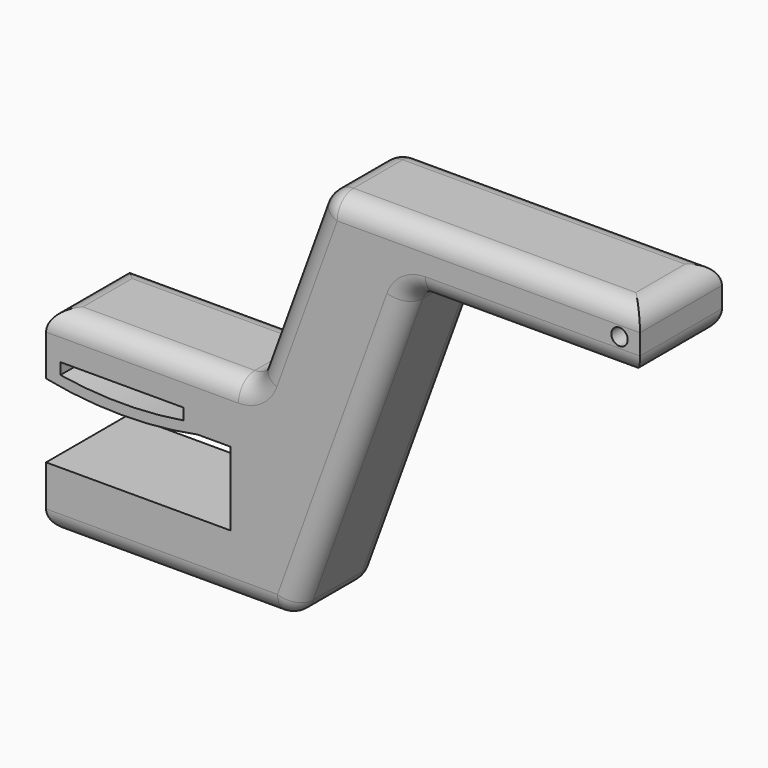
from build123d import *

# Parameters (mm, degrees)
F1_DEPTH = 25
F2_F1_R  = 5
F2_F2_R  = 5
F3_R     = 2
F4_DEPTH = 25


with BuildPart() as f1:
    # F0 (on Front) → F1 (new body)
    with BuildSketch(Plane.XZ):
        with BuildLine():
            Line((45, 15), (0, 15))
            Line((0, 15), (0, 0))
            Line((0, 0), (60, 0))
            Line((60, 0), (89.1176187413, 80))
            Line((89.1176187413, 80), (145, 80))
            Line((145, 80), (145, 95))
            Line((145, 95), (67.5712870168, 95))
            Line((67.5712870168, 95), (50.4646860063, 48))
            Line((50.4646860063, 48), (0, 48))
            Line((0, 48), (0, 33))
            ThreePointArc((0, 33), (18.5, 31.181274943), (37, 33))
            Line((37, 33), (45, 33))
            Line((45, 33), (45, 15))
        make_face()
        with BuildLine():
            ThreePointArc((33.5, 34.9055936253), (18.5, 33.681274943), (3.5, 34.9055936253))
            Line((3.5, 34.9055936253), (3.5, 37.681274943))
            Line((3.5, 37.681274943), (33.5, 37.681274943))
            Line((33.5, 37.681274943), (33.5, 34.9055936253))
        make_face(mode=Mode.SUBTRACT)
    extrude(amount=F1_DEPTH)

    # F2: fillet of radius 5 on 16 edges, made by hand

    # F2_f1
    f2_f1_edges = [f1.edges().sort_by_distance(p)[0] for p in [
        (89.1176187413, -12.5, 80),
        (50.4646860063, -12.5, 48),
    ]]
    fillet(f2_f1_edges, radius=F2_F1_R)

    # F2_f2
    f2_f2_edges = [f1.edges().sort_by_distance(p)[0] for p in [
        (60, -12.5, 0),
        (67.5712870168, -12.5, 95),
        (145, -12.5, 95),
        (145, -12.5, 80),
        (0, -12.5, 48),
        (0, -12.5, 0),
        (118.8093282162, -25, 80),
        (73.9600966642, 0, 38.3550503583),
        (106.2856435084, -25, 95),
        (59.616699218, -25, 73.1449496417),
        (106.2856435084, 0, 95),
        (59.616699218, 0, 73.1449496417),
        (30, -25, 0),
        (30, 0, 0),
        (49.831530497, 0, 48.9042397786),
        (49.831530497, -25, 48.9042397786),
        (89.7507742506, 0, 79.0957602214),
        (89.7507742506, -25, 79.0957602214),
    ]]
    fillet(f2_f2_edges, radius=F2_F2_R)

    # F3 (on face) → F4 (cut)
    with BuildSketch(Plane.XZ.offset(25)):
        with Locations((140, 87.5)):
            Circle(F3_R)
    extrude(amount=-F4_DEPTH, mode=Mode.SUBTRACT)


solid = f1.part
